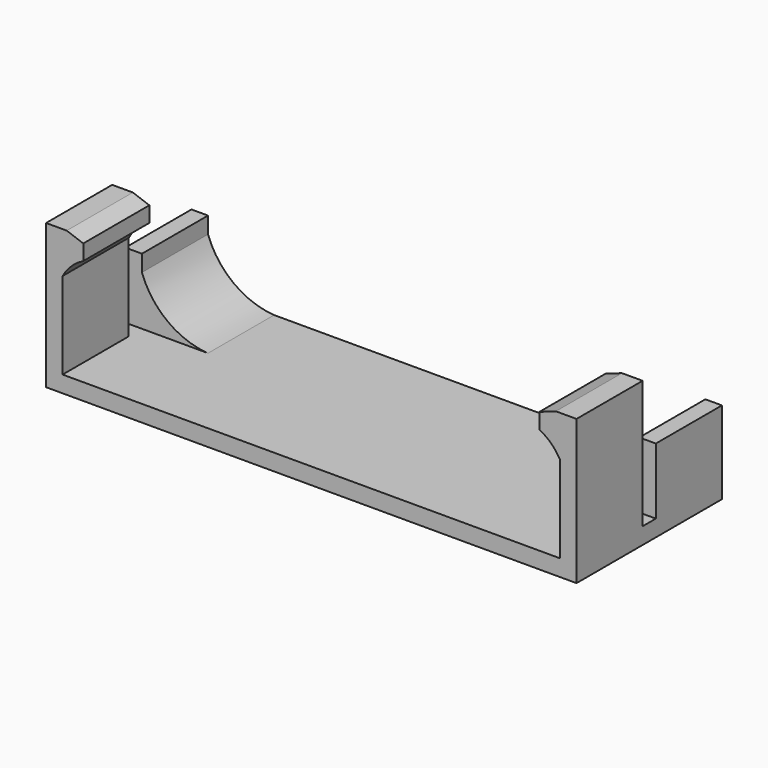
from build123d import *

# Parameters (mm, degrees)
F1_DEPTH = 10
F2_DEPTH = 12
F4_DEPTH = 10


# Not quite as in the source:
# - ends of sketch curves that miss each other by under 0.0002 mm in the source are joined


with BuildPart() as f1:
    # F0 (on Front) → F1 (new body)
    with BuildSketch(Plane.XZ):
        Polygon((0, 2), (0, 0), (64.2, 0), (64.2, 2), (62.2, 2), (2, 2), align=None)
        with BuildLine():
            Line((0, 17.5), (0, 2))
            Line((0, 2), (2, 2))
            Line((2, 2), (2, 12.5))
            ThreePointArc((2, 12.5), (3.0649650296, 13.8955071669), (4.5, 14.9065785791))
            Line((4.5, 14.9065785791), (4.5, 16.7855147476))
            Line((4.5, 16.7855147476), (2.5, 17.5))
            Line((2.5, 17.5), (0, 17.5))
        make_face()
        with BuildLine():
            Line((62.2, 2), (64.2, 2))
            Line((64.2, 2), (64.2, 17.5))
            Line((64.2, 17.5), (61.7, 17.5))
            Line((61.7, 17.5), (59.7, 16.7855148221))
            Line((59.7, 16.7855148221), (59.7, 14.9065787654))
            ThreePointArc((59.7, 14.9065787654), (61.1350349704, 13.8955073531), (62.2, 12.5000001863))
            Line((62.2, 12.5000001863), (62.2, 2))
        make_face()
    extrude(amount=F1_DEPTH)

    # F0 (on Front) → F2 (join)
    with BuildSketch(Plane.XZ):
        Polygon((0, 2), (0, 0), (64.2, 0), (64.2, 2), (62.2, 2), (2, 2), align=None)
    extrude(amount=-F2_DEPTH)

    # F3 (on face) → F4 (join)
    with BuildSketch(Plane(origin=(0, 12, 0), x_dir=(-1, 0, 0), z_dir=(0, 1, 0))):
        with BuildLine():
            Line((-64.2, 2), (-54.2, 2))
            ThreePointArc((-54.2, 2), (-59.0968473433, 3.8042035422), (-62.2, 8))
            Line((-62.2, 8), (-62.2, 10))
            Line((-62.2, 10), (-64.2, 10))
            Line((-64.2, 10), (-64.2, 2))
        make_face()
        with BuildLine():
            Line((-10, 2), (0, 2))
            Line((0, 2), (0, 10))
            Line((0, 10), (-2, 10))
            Line((-2, 10), (-2, 8))
            ThreePointArc((-2, 8), (-5.1031526567, 3.8042035422), (-10, 2))
        make_face()
    extrude(amount=-F4_DEPTH)


solid = f1.part
